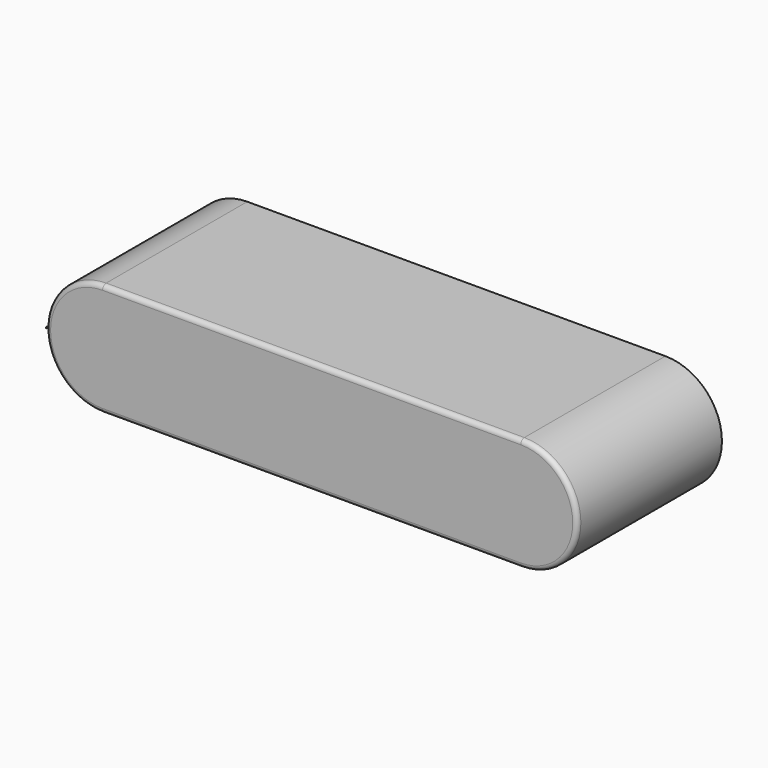
from build123d import *
from build123d import SkipClean  # not in build123d's __all__

# Parameters (mm, degrees)
F1_DEPTH    = 800
F2_T1_DEPTH = 1850
F2_T4_ANGLE = 180
F2_T6_ANGLE = 90
F2_T8_ANGLE = 90


# Not quite as in the source:
# - a fillet or chamfer that OpenCascade refuses, or shapes differently, is made with other operations: its cross-section is extruded or revolved along the edge and cut away or added


with BuildPart() as f1:
    # F0 (on Front) → F1 (new body)
    with BuildSketch(Plane.XZ):
        with BuildLine():
            ThreePointArc((-2350, 255.7604187137), (-2350.0164017124, 252.8802093568), (-2350, 250))
            Line((-2350, 250), (-2350, 255.7604187137))
        make_face()
        with BuildLine():
            Line((-2100, 0), (-250, 0))
            ThreePointArc((-250, 0), (0, 250), (-250, 500))
            Line((-250, 500), (-2100, 500))
            ThreePointArc((-2100, 500), (-2276.7766952966, 426.7766952966), (-2350, 250))
            ThreePointArc((-2350, 250), (-2276.7766952966, 73.2233047034), (-2100, 0))
        make_face()
    extrude(amount=F1_DEPTH)

    # F2: fillet of radius 20 on 5 edges, made by hand

    # F2_s2 → F2_t1 (cut)
    with BuildSketch(Plane.YZ.offset(-2100)):
        with BuildLine():
            ThreePointArc((-780, 0), (-794.1421356237, 5.8578643763), (-800, 20))
            Line((-800, 20), (-800, 0))
            Line((-800, 0), (-780, 0))
        make_face()
        with BuildLine():
            ThreePointArc((-800, 480), (-794.1421356237, 494.1421356237), (-780, 500))
            Line((-780, 500), (-800, 500))
            Line((-800, 500), (-800, 480))
        make_face()
    extrude(amount=F2_T1_DEPTH, mode=Mode.SUBTRACT)

    # F2_s3 → F2_t4 (revolve, cut)
    with BuildSketch(Plane.YZ.offset(-250)):
        with BuildLine():
            ThreePointArc((-780, 0), (-794.1421356237, 5.8578643763), (-800, 20))
            Line((-800, 20), (-800, 0))
            Line((-800, 0), (-780, 0))
        make_face()
    revolve(axis=Axis((-250, -800, 250), (0, -1, 0)), revolution_arc=F2_T4_ANGLE, mode=Mode.SUBTRACT)

    # F2_s5 → F2_t6 (revolve, cut)
    with BuildSketch(Plane.YZ.offset(-2100)):
        with BuildLine():
            ThreePointArc((-780, 0), (-794.1421356237, 5.8578643763), (-800, 20))
            Line((-800, 20), (-800, 0))
            Line((-800, 0), (-780, 0))
        make_face()
    revolve(axis=Axis((-2100, -800, 250), (0, 1, 0)), revolution_arc=F2_T6_ANGLE, mode=Mode.SUBTRACT)

    # F2_s7 → F2_t8 (revolve, cut)
    with BuildSketch(Plane.XY.offset(250)):
        with BuildLine():
            ThreePointArc((-2330, -800), (-2344.1421356237, -794.1421356237), (-2350, -780))
            Line((-2350, -780), (-2350, -800))
            Line((-2350, -800), (-2330, -800))
        make_face()
    with SkipClean():  # cleaning this boolean's faces spoils the solid; the shape is the same uncleaned
        revolve(axis=Axis((-2100, -800, 250), (0, 1, 0)), revolution_arc=F2_T8_ANGLE, mode=Mode.SUBTRACT)


solid = f1.part
